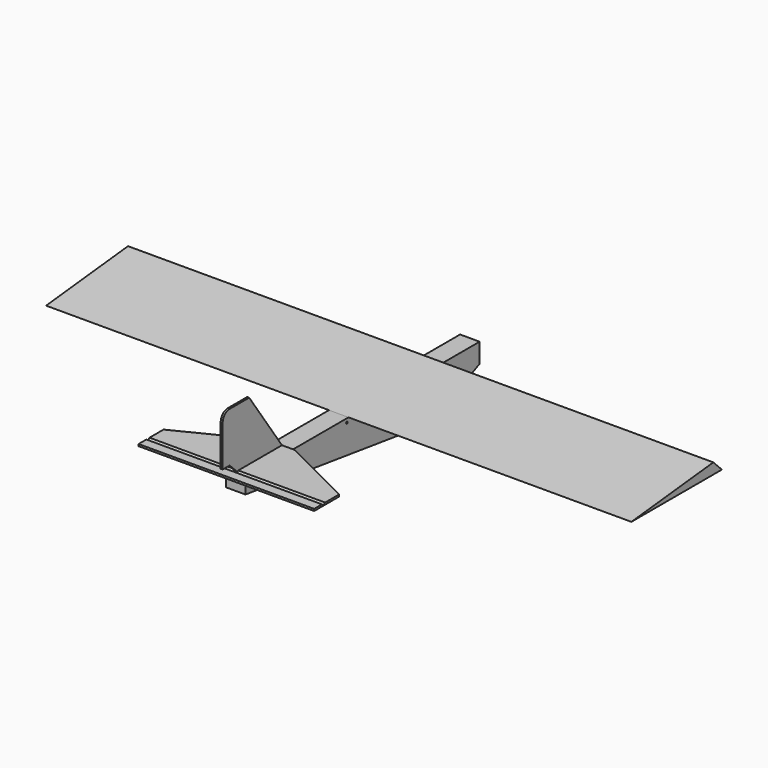
from build123d import *

# Parameters (mm, degrees)
F1_DEPTH = 2.5
F0_R     = 2.5
F2_DEPTH = 25
F3_DEPTH = 225
F5_DEPTH = 25
F6_DEPTH = 750


with BuildPart() as f1:
    # F0 (on Right) → F1 (new body, symmetric)
    with BuildSketch(Plane.YZ):
        with BuildLine():
            Line((-772.5, 137.5), (-750, 115))
            Line((-750, 115), (-750, 265))
            Line((-750, 265), (-772.5, 265))
            ThreePointArc((-772.5, 265), (-788.4099025767, 258.4099025767), (-795, 242.5))
            Line((-795, 242.5), (-795, 137.5))
            Line((-795, 137.5), (-772.5, 137.5))
        make_face()
        Polygon((-750, 115), (-750, 110), (-745, 115), (-605, 115), (-710.0311307315, 265), (-750, 265), align=None)
    extrude(amount=F1_DEPTH, both=True)


with BuildPart() as f2:
    # F0 (on Right) → F2 (new body, symmetric)
    with BuildSketch(Plane.YZ):
        Polygon((-180, 0), (-130, 0), (0, 60), (0, 110), (-130, 110), (-420, 110), (-605, 110), (-750, 110), (-750, 70), (-230, 0), align=None)
        with Locations((-425, 100)):
            Circle(F0_R, mode=Mode.SUBTRACT)
        with Locations((-125, 100)):
            Circle(F0_R, mode=Mode.SUBTRACT)
    extrude(amount=F2_DEPTH, both=True)

    # F0 (on Right) → F6 (join, symmetric)
    with BuildSketch(Plane.YZ):
        Polygon((-420, 110), (-130, 110), (-157.5813151867, 137.5813151867), align=None)
    extrude(amount=F6_DEPTH, both=True)


with BuildPart() as f3:
    # F0 (on Right) → F3 (new body, symmetric)
    with BuildSketch(Plane.YZ):
        Polygon((-780, 110), (-750, 110), (-755, 115), (-780, 115), align=None)
    extrude(amount=F3_DEPTH, both=True)


with BuildPart() as f3b:
    # F0 (on Right) → F3, piece 2 (new body, symmetric)
    with BuildSketch(Plane.YZ):
        Polygon((-745, 115), (-750, 110), (-605, 110), (-605, 115), align=None)
    extrude(amount=F3_DEPTH, both=True)

    # F4 (on face) → F5 (cut)
    with BuildSketch(Plane(origin=(0, 0, 110), x_dir=(1, 0, 0), z_dir=(0, 0, -1))):
        Polygon((225, 605), (225, 700), (35, 605), align=None)
        Polygon((-35, 605), (-225, 700), (-225, 605), align=None)
    extrude(amount=-F5_DEPTH, mode=Mode.SUBTRACT)


solid = Compound([f1.part, f2.part, f3.part, f3b.part])
